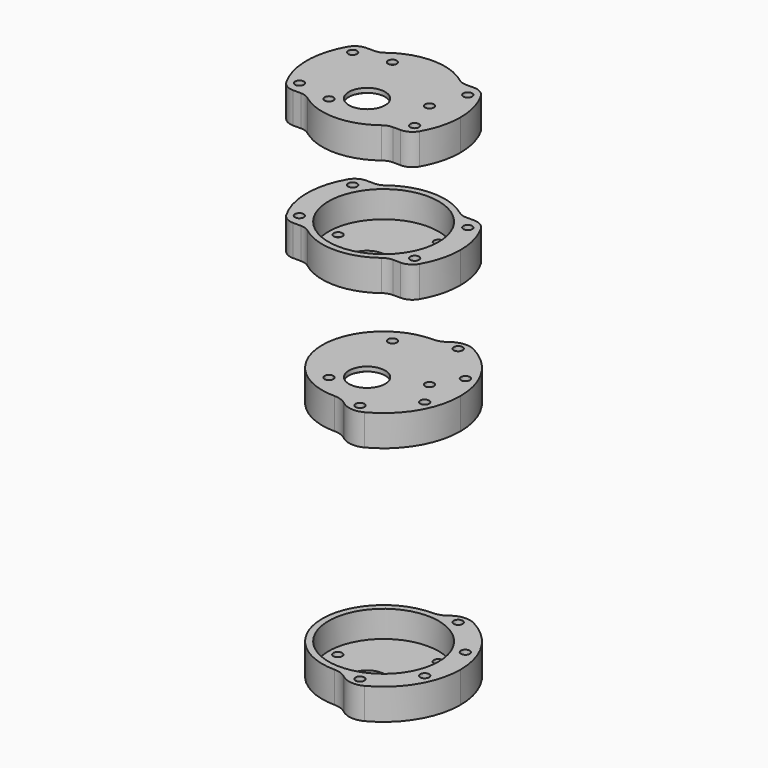
from build123d import *

# Parameters (mm, degrees)
F1_R           = 18.625
F1_R_2         = 1.5
F1_R_3         = 6.125
F3_DEPTH       = 1.5
F2_R           = 18.625
F2_R_2         = 1.5
F2_R_3         = 6.125
F4_DEPTH       = 1.5
F5_DEPTH       = 10.5
F6_DEPTH       = 10.5
F7_T4_DEPTH    = 50.8144607383
F7_S5_R        = 20.75
F7_T6_DEPTH    = 27
F7_T10_DEPTH   = 50.8144607383
F7_S11_R       = 20.75
F7_T12_DEPTH   = 27
F7_2_T4_DEPTH  = 50.8144607383
F7_2_S5_R      = 20.75
F7_2_T6_DEPTH  = 27
F7_2_T10_DEPTH = 50.8144607383
F7_2_S11_R     = 20.75
F7_2_T12_DEPTH = 27
F8_R           = 7
F8_2_R         = 7
F11_R          = 18.625
F11_R_2        = 1.5
F11_R_3        = 6.125
F13_DEPTH      = 1.5
F14_DEPTH      = 10.5
F12_R          = 18.625
F12_R_2        = 1.5
F12_R_3        = 6.125
F15_DEPTH      = 1.5
F16_DEPTH      = 10.5
F17_R          = 5
F17_2_R        = 5


# Not quite as in the source:
# - a fillet or chamfer that OpenCascade refuses, or shapes differently, is made with other operations: its cross-section is extruded or revolved along the edge and cut away or added


with BuildPart() as f3:
    # F1 (on Top) → F3 (new body)
    with BuildSketch(Plane.XY):
        Circle(F1_R)
        with Locations((7.75, -13.4233937587)):
            Circle(F1_R_2, mode=Mode.SUBTRACT)
        with Locations((0, -7)):
            Circle(F1_R_3, mode=Mode.SUBTRACT)
        with Locations((-15.5, 0)):
            Circle(F1_R_2, mode=Mode.SUBTRACT)
        with Locations((7.75, 13.4233937587)):
            Circle(F1_R_2, mode=Mode.SUBTRACT)
    extrude(amount=F3_DEPTH)

    # F1 (on Top) → F5 (join)
    with BuildSketch(Plane.XY):
        with BuildLine():
            ThreePointArc((20.75, 0), (14.6724657096, 14.6724657096), (0, 20.75))
            ThreePointArc((0, 20.75), (-20.75, 0), (0, -20.75))
            ThreePointArc((0, -20.75), (14.6724657096, -14.6724657096), (20.75, 0))
        make_face()
        Circle(F1_R, mode=Mode.SUBTRACT)
        with BuildLine():
            ThreePointArc((0, -26), (18.3847763109, -18.3847763109), (26, 0))
            ThreePointArc((26, 0), (18.3847763109, 18.3847763109), (0, 26))
            Line((0, 26), (0, 20.75))
            ThreePointArc((0, 20.75), (14.6724657096, 14.6724657096), (20.75, 0))
            ThreePointArc((20.75, 0), (14.6724657096, -14.6724657096), (0, -20.75))
            Line((0, -20.75), (0, -26))
        make_face()
        with Locations((8.6103772282, -20.7872894815)):
            Circle(F1_R_2, mode=Mode.SUBTRACT)
        with Locations((20.7872894815, -8.6103772282)):
            Circle(F1_R_2, mode=Mode.SUBTRACT)
        with Locations((20.7872894815, 8.6103772282)):
            Circle(F1_R_2, mode=Mode.SUBTRACT)
        with Locations((8.6103772282, 20.7872894815)):
            Circle(F1_R_2, mode=Mode.SUBTRACT)
    extrude(amount=F5_DEPTH)

    # F7: chamfer of 6 on 2 edges, made by hand


with BuildPart() as f4:
    # F2 (on offset) → F4 (new body)
    with BuildSketch(Plane.XY.offset(92)):
        Circle(F2_R)
        with Locations((-7.75, -13.4233937587)):
            Circle(F2_R_2, mode=Mode.SUBTRACT)
        with Locations((0, -7)):
            Circle(F2_R_3, mode=Mode.SUBTRACT)
        with Locations((-7.75, 13.4233937587)):
            Circle(F2_R_2, mode=Mode.SUBTRACT)
        with Locations((15.5, 0)):
            Circle(F2_R_2, mode=Mode.SUBTRACT)
    extrude(amount=-F4_DEPTH)

    # F2 (on offset) → F6 (join)
    with BuildSketch(Plane.XY.offset(92)):
        with BuildLine():
            ThreePointArc((20.75, 0), (14.6724657096, 14.6724657096), (0, 20.75))
            ThreePointArc((0, 20.75), (-20.75, 0), (0, -20.75))
            ThreePointArc((0, -20.75), (14.6724657096, -14.6724657096), (20.75, 0))
        make_face()
        Circle(F2_R, mode=Mode.SUBTRACT)
        with BuildLine():
            ThreePointArc((0, -26), (18.3847763109, -18.3847763109), (26, 0))
            ThreePointArc((26, 0), (18.3847763109, 18.3847763109), (0, 26))
            Line((0, 26), (0, 20.75))
            ThreePointArc((0, 20.75), (14.6724657096, 14.6724657096), (20.75, 0))
            ThreePointArc((20.75, 0), (14.6724657096, -14.6724657096), (0, -20.75))
            Line((0, -20.75), (0, -26))
        make_face()
        with Locations((8.6103772282, -20.7872894815)):
            Circle(F2_R_2, mode=Mode.SUBTRACT)
        with Locations((20.7872894815, -8.6103772282)):
            Circle(F2_R_2, mode=Mode.SUBTRACT)
        with Locations((20.7872894815, 8.6103772282)):
            Circle(F2_R_2, mode=Mode.SUBTRACT)
        with Locations((8.6103772282, 20.7872894815)):
            Circle(F2_R_2, mode=Mode.SUBTRACT)
    extrude(amount=-F6_DEPTH)

    # F7#2: chamfer of 6 on 2 edges, made by hand


with BuildPart() as f7_tool2:
    # F7_s3 → F7_t4 (new body)
    with BuildSketch(Plane.XY.offset(-20.1572303692)):
        with BuildLine():
            Line((7.8, 24.8024192368), (0, 19.0787840283))
            Line((0, 19.0787840283), (0, 26))
            ThreePointArc((0, 26), (4.0302519246, 25.6857366923), (7.8, 24.8024192368))
        make_face()
    extrude(amount=F7_T4_DEPTH)

    # F7_s5 → F7_t6 (cut, symmetric)
    with BuildSketch(Plane.XY.offset(5.3)):
        Circle(F7_S5_R)
    extrude(amount=F7_T6_DEPTH, both=True, mode=Mode.SUBTRACT)


with BuildPart() as f3_1:
    add(f3.part)

    # F7_t1: cut F7_tool2
    add(f7_tool2.part, mode=Mode.SUBTRACT)


with BuildPart() as f7_tool8:
    # F7_s9 → F7_t10 (new body)
    with BuildSketch(Plane.XY.offset(-20.1572303692)):
        with BuildLine():
            Line((0, -19.0787840283), (7.8, -24.8024192368))
            ThreePointArc((7.8, -24.8024192368), (4.0302519246, -25.6857366923), (0, -26))
            Line((0, -26), (0, -19.0787840283))
        make_face()
    extrude(amount=F7_T10_DEPTH)

    # F7_s11 → F7_t12 (cut, symmetric)
    with BuildSketch(Plane.XY.offset(5.3)):
        Circle(F7_S11_R)
    extrude(amount=F7_T12_DEPTH, both=True, mode=Mode.SUBTRACT)


with BuildPart() as f3_2:
    add(f3_1.part)

    # F7_t7: cut F7_tool8
    add(f7_tool8.part, mode=Mode.SUBTRACT)

    # F8
    f8_edges = [f3_2.edges().sort_by_distance(p)[0] for p in [
        (2.12834, -20.640559, 5.25),
        (2.12834, 20.640559, 5.25),
        (7.8, 24.802419, 5.25),
        (7.8, -24.802419, 5.25),
    ]]
    fillet(f8_edges, radius=F8_R)


with BuildPart() as f7_2_tool2:
    # F7_2_s3 → F7_2_t4 (new body)
    with BuildSketch(Plane.XY.offset(112.1572303692)):
        with BuildLine():
            Line((7.8, 24.8024192368), (0, 19.0787840283))
            Line((0, 19.0787840283), (0, 26))
            ThreePointArc((0, 26), (4.0302519246, 25.6857366923), (7.8, 24.8024192368))
        make_face()
    extrude(amount=-F7_2_T4_DEPTH)

    # F7_2_s5 → F7_2_t6 (cut, symmetric)
    with BuildSketch(Plane.XY.offset(86.8)):
        Circle(F7_2_S5_R)
    extrude(amount=F7_2_T6_DEPTH, both=True, mode=Mode.SUBTRACT)


with BuildPart() as f4_1:
    add(f4.part)

    # F7_2_t1: cut F7_2_tool2
    add(f7_2_tool2.part, mode=Mode.SUBTRACT)


with BuildPart() as f7_2_tool8:
    # F7_2_s9 → F7_2_t10 (new body)
    with BuildSketch(Plane.XY.offset(112.1572303692)):
        with BuildLine():
            Line((0, -19.0787840283), (7.8, -24.8024192368))
            ThreePointArc((7.8, -24.8024192368), (4.0302519246, -25.6857366923), (0, -26))
            Line((0, -26), (0, -19.0787840283))
        make_face()
    extrude(amount=-F7_2_T10_DEPTH)

    # F7_2_s11 → F7_2_t12 (cut, symmetric)
    with BuildSketch(Plane.XY.offset(86.8)):
        Circle(F7_2_S11_R)
    extrude(amount=F7_2_T12_DEPTH, both=True, mode=Mode.SUBTRACT)


with BuildPart() as f4_2:
    add(f4_1.part)

    # F7_2_t7: cut F7_2_tool8
    add(f7_2_tool8.part, mode=Mode.SUBTRACT)

    # F8#2
    f8_2_edges = [f4_2.edges().sort_by_distance(p)[0] for p in [
        (7.8, -24.802419, 86.75),
        (2.12834, -20.640559, 86.75),
        (2.12834, 20.640559, 86.75),
        (7.8, 24.802419, 86.75),
    ]]
    fillet(f8_2_edges, radius=F8_2_R)


with BuildPart() as f13:
    # F11 (on offset) → F13 (new body)
    with BuildSketch(Plane.XY.offset(125)):
        Circle(F11_R)
        with Locations((7.6452526616, -13.4833271762)):
            Circle(F11_R_2, mode=Mode.SUBTRACT)
        with Locations((0, -7)):
            Circle(F11_R_3, mode=Mode.SUBTRACT)
        with Locations((-15.4995301929, 0.1206805648)):
            Circle(F11_R_2, mode=Mode.SUBTRACT)
        with Locations((7.8542775313, 13.3626466114)):
            Circle(F11_R_2, mode=Mode.SUBTRACT)
    extrude(amount=F13_DEPTH)

    # F11 (on offset) → F14 (join)
    with BuildSketch(Plane.XY.offset(125)):
        with BuildLine():
            Line((-13.7953796613, 15.5), (-20.8746257451, 15.5))
            ThreePointArc((-20.8746257451, 15.5), (-26, 0), (-20.8746257451, -15.5))
            Line((-20.8746257451, -15.5), (-13.7953796613, -15.5))
            ThreePointArc((-13.7953796613, -15.5), (-20.75, 0), (-13.7953796613, 15.5))
        make_face()
        with Locations((-19.4855715851, -11.25)):
            Circle(F11_R_2, mode=Mode.SUBTRACT)
        with Locations((-19.4855715851, 11.25)):
            Circle(F11_R_2, mode=Mode.SUBTRACT)
        with BuildLine():
            ThreePointArc((20.75, 0), (18.9316748859, 8.4943620133), (13.7953796613, 15.5))
            ThreePointArc((13.7953796613, 15.5), (0, 20.75), (-13.7953796613, 15.5))
            ThreePointArc((-13.7953796613, 15.5), (-20.75, 0), (-13.7953796613, -15.5))
            ThreePointArc((-13.7953796613, -15.5), (0, -20.75), (13.7953796613, -15.5))
            ThreePointArc((13.7953796613, -15.5), (18.9316748859, -8.4943620133), (20.75, 0))
        make_face()
        Circle(F11_R, mode=Mode.SUBTRACT)
        with BuildLine():
            ThreePointArc((20.8746257451, -15.5), (24.6854235266, -8.1627118847), (26, 0))
            ThreePointArc((26, 0), (24.6854235266, 8.1627118847), (20.8746257451, 15.5))
            Line((20.8746257451, 15.5), (13.7953796613, 15.5))
            ThreePointArc((13.7953796613, 15.5), (18.9316748859, 8.4943620133), (20.75, 0))
            ThreePointArc((20.75, 0), (18.9316748859, -8.4943620133), (13.7953796613, -15.5))
            Line((13.7953796613, -15.5), (20.8746257451, -15.5))
        make_face()
        with Locations((19.4855715851, -11.25)):
            Circle(F11_R_2, mode=Mode.SUBTRACT)
        with Locations((19.4855715851, 11.25)):
            Circle(F11_R_2, mode=Mode.SUBTRACT)
    extrude(amount=F14_DEPTH)

    # F17
    f17_edges = [f13.edges().sort_by_distance(p)[0] for p in [
        (13.79538, 15.5, 130.25),
        (13.79538, -15.5, 130.25),
        (-13.79538, -15.5, 130.25),
        (-13.79538, 15.5, 130.25),
        (-20.874626, -15.5, 130.25),
        (20.874626, -15.5, 130.25),
        (20.874626, 15.5, 130.25),
        (-20.874626, 15.5, 130.25),
    ]]
    fillet(f17_edges, radius=F17_R)


with BuildPart() as f15:
    # F12 (on offset) → F15 (new body)
    with BuildSketch(Plane.XY.offset(175)):
        Circle(F12_R)
        with Locations((-7.75, -13.4233937587)):
            Circle(F12_R_2, mode=Mode.SUBTRACT)
        with Locations((0, -7)):
            Circle(F12_R_3, mode=Mode.SUBTRACT)
        with Locations((-7.75, 13.4233937587)):
            Circle(F12_R_2, mode=Mode.SUBTRACT)
        with Locations((15.5, 0)):
            Circle(F12_R_2, mode=Mode.SUBTRACT)
    extrude(amount=-F15_DEPTH)

    # F12 (on offset) → F16 (join)
    with BuildSketch(Plane.XY.offset(175)):
        with BuildLine():
            ThreePointArc((20.8746257451, -15.5), (24.6854235266, -8.1627118847), (26, 0))
            ThreePointArc((26, 0), (24.6854235266, 8.1627118847), (20.8746257451, 15.5))
            Line((20.8746257451, 15.5), (13.7953796613, 15.5))
            ThreePointArc((13.7953796613, 15.5), (18.9316748859, 8.4943620133), (20.75, 0))
            ThreePointArc((20.75, 0), (18.9316748859, -8.4943620133), (13.7953796613, -15.5))
            Line((13.7953796613, -15.5), (20.8746257451, -15.5))
        make_face()
        with Locations((19.4855715851, -11.25)):
            Circle(F12_R_2, mode=Mode.SUBTRACT)
        with Locations((19.4855715851, 11.25)):
            Circle(F12_R_2, mode=Mode.SUBTRACT)
        with BuildLine():
            ThreePointArc((20.75, 0), (18.9316748859, 8.4943620133), (13.7953796613, 15.5))
            ThreePointArc((13.7953796613, 15.5), (0, 20.75), (-13.7953796613, 15.5))
            ThreePointArc((-13.7953796613, 15.5), (-20.75, 0), (-13.7953796613, -15.5))
            ThreePointArc((-13.7953796613, -15.5), (0, -20.75), (13.7953796613, -15.5))
            ThreePointArc((13.7953796613, -15.5), (18.9316748859, -8.4943620133), (20.75, 0))
        make_face()
        Circle(F12_R, mode=Mode.SUBTRACT)
        with BuildLine():
            Line((-13.7953796613, 15.5), (-20.8746257451, 15.5))
            ThreePointArc((-20.8746257451, 15.5), (-26, 0), (-20.8746257451, -15.5))
            Line((-20.8746257451, -15.5), (-13.7953796613, -15.5))
            ThreePointArc((-13.7953796613, -15.5), (-20.75, 0), (-13.7953796613, 15.5))
        make_face()
        with Locations((-19.4855715851, -11.25)):
            Circle(F12_R_2, mode=Mode.SUBTRACT)
        with Locations((-19.4855715851, 11.25)):
            Circle(F12_R_2, mode=Mode.SUBTRACT)
    extrude(amount=-F16_DEPTH)

    # F17#2
    f17_2_edges = [f15.edges().sort_by_distance(p)[0] for p in [
        (-13.79538, 15.5, 169.75),
        (-20.874626, 15.5, 169.75),
        (13.79538, 15.5, 169.75),
        (20.874626, 15.5, 169.75),
        (20.874626, -15.5, 169.75),
        (13.79538, -15.5, 169.75),
        (-13.79538, -15.5, 169.75),
        (-20.874626, -15.5, 169.75),
    ]]
    fillet(f17_2_edges, radius=F17_2_R)


solid = Compound([f3_2.part, f4_2.part, f13.part, f15.part])
